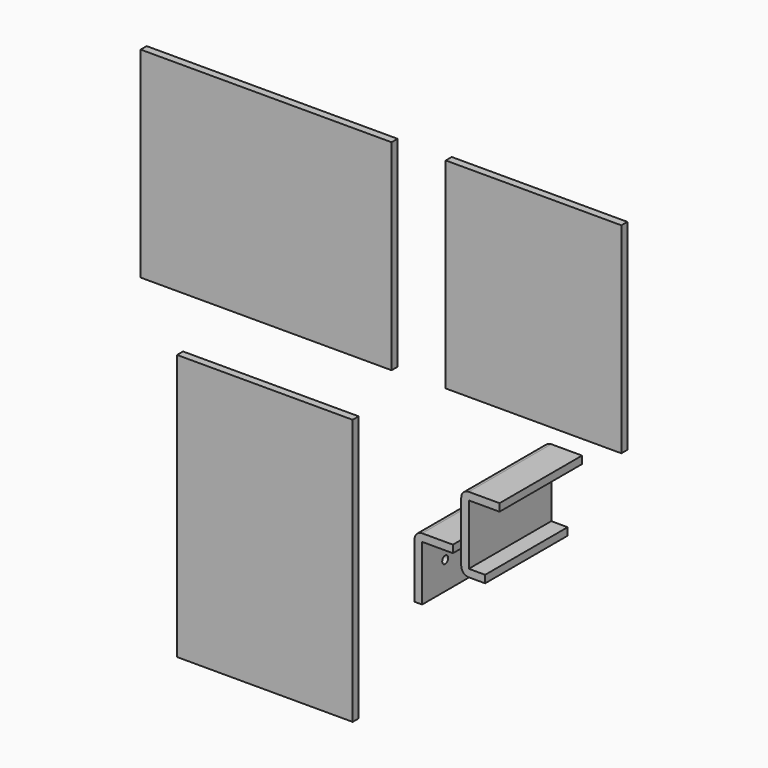
from build123d import *

# Parameters (mm, degrees)
F0_W     = 70
F0_H     = 80
F1_DEPTH = 3
F2_DEPTH = 3
F0_W_2   = 100
F0_H_2   = 106
F3_DEPTH = 20
F4_R     = 1.5
F5_DEPTH = 25.4
F6_DEPTH = 38.1


with BuildPart() as f1:
    # F0 (on Front) → F1 (new body)
    with BuildSketch(Plane.XZ):
        with Locations((20.1463365555, 12.1699897945)):
            Rectangle(F0_W, F0_H)
    extrude(amount=F1_DEPTH)

    # F0 (on Front) → F2 (join)
    with BuildSketch(Plane.XZ):
        with Locations((20.1463365555, 12.1699897945)):
            Rectangle(F0_W, F0_H)
    extrude(amount=F2_DEPTH)


with BuildPart() as f2:
    # F0 (on Front) → F2, piece 2 (new body)
    with BuildSketch(Plane.XZ):
        with Locations((-86.4454574883, 11.532458514)):
            Rectangle(F0_W_2, F0_H)
    extrude(amount=F2_DEPTH)


with BuildPart() as f2b:
    # F0 (on Front) → F2, piece 3 (new body)
    with BuildSketch(Plane.XZ):
        with Locations((-86.9487600029, -103.8902209401)):
            Rectangle(F0_W, F0_H_2)
    extrude(amount=F2_DEPTH)


with BuildPart() as f2c:
    # F0 (on Front) → F2, piece 4 (new body)
    with BuildSketch(Plane.XZ):
        with BuildLine():
            Line((-11.2519366667, -71.3728516102), (-11.2519366667, -93.3728516102))
            Line((-11.2519366667, -93.3728516102), (-8.2519366667, -93.3728516102))
            Line((-8.2519366667, -93.3728516102), (-8.2519366667, -71.3728516102))
            Line((-8.2519366667, -71.3728516102), (4.0119807236, -71.3728516102))
            Line((4.0119807236, -71.3728516102), (4.0119807236, -68.3728516102))
            Line((4.0119807236, -68.3728516102), (-8.2519366667, -68.3728516102))
            ThreePointArc((-8.2519366667, -68.3728516102), (-10.3732570102, -69.2515312666), (-11.2519366667, -71.3728516102))
        make_face()
    extrude(amount=F2_DEPTH)

    # F3 (add): a face of the model
    f3_faces = [f2c.faces().sort_by_distance(p)[0] for p in [
        (-8.5448508476, -3, -82.3728516102),
    ]]
    extrude(f3_faces, amount=F3_DEPTH)

    # F4 (on Right) → F5 (cut)
    with BuildSketch(Plane.YZ):
        with Locations((-11.4885549992, -82.3099240661)):
            Circle(F4_R)
    extrude(amount=-F5_DEPTH, mode=Mode.SUBTRACT)


with BuildPart() as f2d:
    # F0 (on Front) → F2, piece 5 (new body)
    with BuildSketch(Plane.XZ):
        with BuildLine():
            Line((37.0798228342, -38.7036602497), (37.0798228342, -35.7036602497))
            Line((37.0798228342, -35.7036602497), (24.8158960342, -35.7036602497))
            ThreePointArc((24.8158960342, -35.7036602497), (22.6945756907, -36.5823399062), (21.8158960342, -38.7036602497))
            Line((21.8158960342, -38.7036602497), (21.8158960342, -62.7036602497))
            ThreePointArc((21.8158960342, -62.7036602497), (22.6945756907, -64.8249805933), (24.8158960342, -65.7036602497))
            Line((24.8158960342, -65.7036602497), (31.3320420682, -65.7036602497))
            Line((31.3320420682, -65.7036602497), (31.3320420682, -62.7036602497))
            Line((31.3320420682, -62.7036602497), (24.8158960342, -62.7036602497))
            Line((24.8158960342, -62.7036602497), (24.8158960342, -38.7036602497))
            Line((24.8158960342, -38.7036602497), (37.0798228342, -38.7036602497))
        make_face()
    extrude(amount=F2_DEPTH)

    # F6 (add): a face of the model
    f6_faces = [f2d.faces().sort_by_distance(p)[0] for p in [
        (36.7432240432, -3, -37.2036602497),
    ]]
    extrude(f6_faces, amount=F6_DEPTH)


solid = Compound([f1.part, f2.part, f2b.part, f2c.part, f2d.part])
